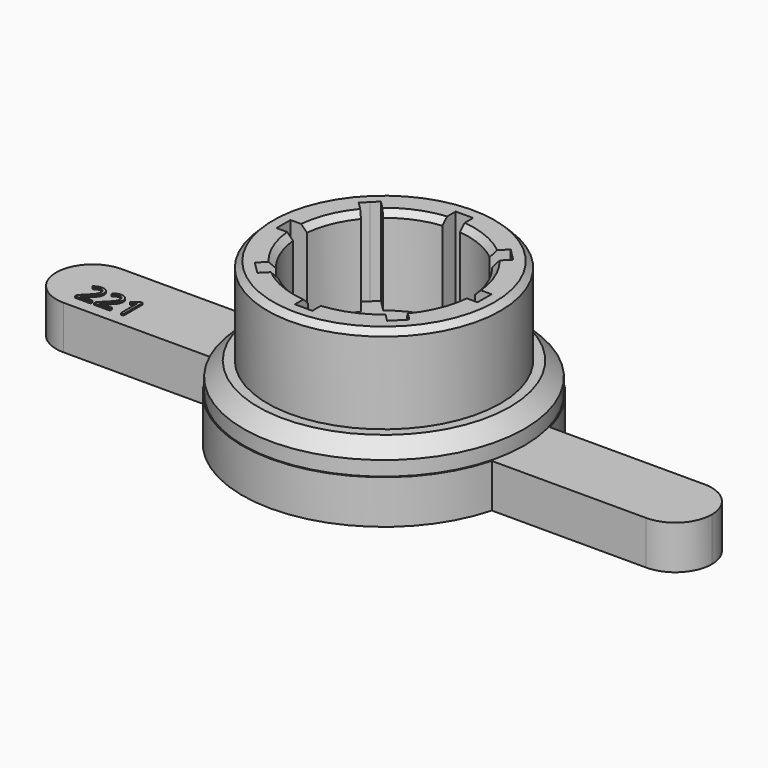
from build123d import *

# Parameters (mm, degrees)
F0_R         = 40
F1_DEPTH     = 30
F2_R         = 48.233355844
F3_DEPTH     = 10
F5_DEPTH     = 15
F6_SIZE      = 2
F7_SIZE      = 2
F8_SIZE      = 5
F9_TEXT_SIZE = 11.5566046184
F10_DEPTH    = 0.5


# Not quite as in the source:
# - a feature names something its author has since deleted; it is built from what else it names
# - Text() gives the source's letters only with a copy of the font that has no kerning and outlines rounded to 1/6400 em; it was checked with that copy


with BuildPart() as f1:
    # F0 (on Top) → F1 (new body)
    with BuildSketch(Plane.XY):
        Circle(F0_R)
        with BuildLine():
            ThreePointArc((22.5173983979, 18.2747577108), (26.7925064428, 11.0978195386), (28.8444102037, 3))
            Line((28.8444102037, 3), (34.5, 3))
            Line((34.5, 3), (34.5, 0))
            Line((34.5, 0), (34.5, -3))
            Line((34.5, -3), (28.8444102037, -3))
            ThreePointArc((28.8444102037, -3), (26.7925064428, -11.0978195386), (22.5173983979, -18.2747577108))
            Line((22.5173983979, -18.2747577108), (26.5165042945, -22.2738636074))
            Line((26.5165042945, -22.2738636074), (24.3951839509, -24.3951839509))
            Line((24.3951839509, -24.3951839509), (22.2738636074, -26.5165042945))
            Line((22.2738636074, -26.5165042945), (18.2747577108, -22.5173983979))
            ThreePointArc((18.2747577108, -22.5173983979), (11.0978195386, -26.7925064428), (3, -28.8444102037))
            Line((3, -28.8444102037), (3, -34.5))
            Line((3, -34.5), (0, -34.5))
            Line((0, -34.5), (-3, -34.5))
            Line((-3, -34.5), (-3, -28.8444102037))
            ThreePointArc((-3, -28.8444102037), (-11.0978195386, -26.7925064428), (-18.2747577108, -22.5173983979))
            Line((-18.2747577108, -22.5173983979), (-22.2738636074, -26.5165042945))
            Line((-22.2738636074, -26.5165042945), (-24.3951839509, -24.3951839509))
            Line((-24.3951839509, -24.3951839509), (-26.5165042945, -22.2738636074))
            Line((-26.5165042945, -22.2738636074), (-22.5173983979, -18.2747577108))
            ThreePointArc((-22.5173983979, -18.2747577108), (-26.7925064428, -11.0978195386), (-28.8444102037, -3))
            Line((-28.8444102037, -3), (-34.5, -3))
            Line((-34.5, -3), (-34.5, 0))
            Line((-34.5, 0), (-34.5, 3))
            Line((-34.5, 3), (-28.8444102037, 3))
            ThreePointArc((-28.8444102037, 3), (-26.7925064428, 11.0978195386), (-22.5173983979, 18.2747577108))
            Line((-22.5173983979, 18.2747577108), (-26.5165042945, 22.2738636074))
            Line((-26.5165042945, 22.2738636074), (-24.3951839509, 24.3951839509))
            Line((-24.3951839509, 24.3951839509), (-22.2738636074, 26.5165042945))
            Line((-22.2738636074, 26.5165042945), (-18.2747577108, 22.5173983979))
            ThreePointArc((-18.2747577108, 22.5173983979), (-11.0978195386, 26.7925064428), (-3, 28.8444102037))
            Line((-3, 28.8444102037), (-3, 34.5))
            Line((-3, 34.5), (0, 34.5))
            Line((0, 34.5), (3, 34.5))
            Line((3, 34.5), (3, 28.8444102037))
            ThreePointArc((3, 28.8444102037), (11.0978195386, 26.7925064428), (18.2747577108, 22.5173983979))
            Line((18.2747577108, 22.5173983979), (22.2738636074, 26.5165042945))
            Line((22.2738636074, 26.5165042945), (24.3951839509, 24.3951839509))
            Line((24.3951839509, 24.3951839509), (26.5165042945, 22.2738636074))
            Line((26.5165042945, 22.2738636074), (22.5173983979, 18.2747577108))
        make_face(mode=Mode.SUBTRACT)
    extrude(amount=F1_DEPTH)

    # F2 (on Top) → F3 (join)
    with BuildSketch(Plane.XY):
        Circle(F2_R)
    extrude(amount=-F3_DEPTH)

    # F4 (on face) → F5 (join)
    with BuildSketch(Plane(origin=(0, 0, -10), x_dir=(1, 0, 0), z_dir=(0, 0, -1))):
        with BuildLine():
            ThreePointArc((100, 12.5), (87.5, 0), (100, -12.5))
            Line((100, -12.5), (100, 12.5))
        make_face()
        with BuildLine():
            Line((46.9918923323, -12.5), (100, -12.5))
            ThreePointArc((100, -12.5), (87.5, 0), (100, 12.5))
            Line((100, 12.5), (46.9918923323, 12.5))
            ThreePointArc((46.9918923323, 12.5), (48.2157429418, 6.3031799551), (48.6260007092, 0))
            ThreePointArc((48.6260007092, 0), (48.2157429418, -6.3031799551), (46.9918923323, -12.5))
        make_face()
        with BuildLine():
            Line((100, 12.5), (100, -12.5))
            ThreePointArc((100, -12.5), (108.8388347648, -8.8388347648), (112.5, 0))
            ThreePointArc((112.5, 0), (108.8388347648, 8.8388347648), (100, 12.5))
        make_face()
        with BuildLine():
            ThreePointArc((-46.9918923323, -12.5), (0, -48.6260007092), (46.9918923323, -12.5))
            Line((46.9918923323, -12.5), (-46.9918923323, -12.5))
        make_face()
        with BuildLine():
            Line((-46.9918923323, -12.5), (46.9918923323, -12.5))
            ThreePointArc((46.9918923323, -12.5), (48.2157429418, -6.3031799551), (48.6260007092, 0))
            ThreePointArc((48.6260007092, 0), (48.2157429418, 6.3031799551), (46.9918923323, 12.5))
            Line((46.9918923323, 12.5), (-46.9918923323, 12.5))
            ThreePointArc((-46.9918923323, 12.5), (-48.6260007092, 0), (-46.9918923323, -12.5))
        make_face()
        with BuildLine():
            Line((-100, -12.5), (-46.9918923323, -12.5))
            ThreePointArc((-46.9918923323, -12.5), (-48.6260007092, 0), (-46.9918923323, 12.5))
            Line((-46.9918923323, 12.5), (-100, 12.5))
            ThreePointArc((-100, 12.5), (-91.1611652352, 8.8388347648), (-87.5, 0))
            ThreePointArc((-87.5, 0), (-91.1611652352, -8.8388347648), (-100, -12.5))
        make_face()
        with BuildLine():
            Line((-46.9918923323, 12.5), (46.9918923323, 12.5))
            ThreePointArc((46.9918923323, 12.5), (0, 48.6260007092), (-46.9918923323, 12.5))
        make_face()
        with BuildLine():
            ThreePointArc((-100, 12.5), (-112.5, 0), (-100, -12.5))
            Line((-100, -12.5), (-100, 12.5))
        make_face()
        with BuildLine():
            Line((-100, 12.5), (-100, -12.5))
            ThreePointArc((-100, -12.5), (-91.1611652352, -8.8388347648), (-87.5, 0))
            ThreePointArc((-87.5, 0), (-91.1611652352, 8.8388347648), (-100, 12.5))
        make_face()
    extrude(amount=F5_DEPTH)

    # F6
    f6_edges = [f1.edges().sort_by_distance(p)[0] for p in [
        (-26.792506, 11.09782, 30),
        (-26.792506, -11.09782, 30),
        (-11.09782, -26.792506, 30),
        (11.09782, -26.792506, 30),
        (26.792506, -11.09782, 30),
        (26.792506, 11.09782, 30),
        (11.09782, 26.792506, 30),
        (-11.09782, 26.792506, 30),
    ]]
    chamfer(f6_edges, length=F6_SIZE)

    # F7
    f7_edges = [f1.edges().sort_by_distance(p)[0] for p in [
        (-40, 0, 30),
    ]]
    chamfer(f7_edges, length=F7_SIZE)

    # F8
    f8_edges = [f1.edges().sort_by_distance(p)[0] for p in [
        (-48.233356, 0, 0),
    ]]
    chamfer(f8_edges, length=F8_SIZE)

    # F9 (on face) → F10 (join)
    with BuildSketch(Plane.XY.offset(-10)):
        with Locations((-100, -8.3207553253)):
            Text('221', F9_TEXT_SIZE, font='Open Sans', text_align=(TextAlign.LEFT, TextAlign.BOTTOM))
    extrude(amount=F10_DEPTH)


solid = f1.part
